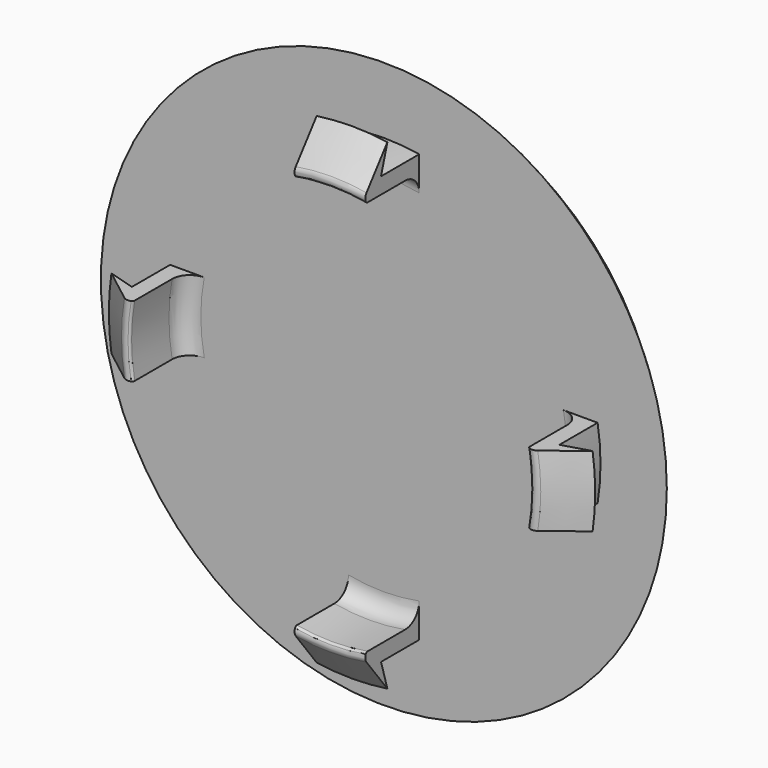
from build123d import *

# Parameters (mm, degrees)
F3_DEPTH      = 32.001
F3_DEPTH_BACK = 32.001
F5_DEPTH      = 32.001
F5_DEPTH_BACK = 32.001


# Not quite as in the source:
# - a feature names something its author has since deleted; it is built from what else it names


with BuildPart() as f1:
    # F0 (on Top) → F1 (revolve)
    with BuildSketch(Plane.XY):
        with BuildLine():
            Line((29, 3), (0, 3))
            Line((0, 3), (0, 0))
            Line((0, 0), (20.7, 0))
            ThreePointArc((20.7, 0), (22.1142135624, -0.5857864376), (22.7, -2))
            Line((22.7, -2), (22.7, -7.2844397868))
            ThreePointArc((22.7, -7.2844397868), (22.7497180358, -7.4498451628), (22.8823929227, -7.5604263361))
            ThreePointArc((22.8823929227, -7.5604263361), (23.3097624273, -7.6192211516), (23.7078530386, -7.45301228))
            Line((23.7078530386, -7.45301228), (27.5, -4.5))
            Line((27.5, -4.5), (24.5, -5.4))
            Line((24.5, -5.4), (24.5, -3))
            Line((24.5, -3), (24.5, 0))
            Line((24.5, 0), (32, 0))
            Line((32, 0), (29, 3))
        make_face()
    revolve(axis=Axis((0, -3.2623065636, 0), (0, -1, 0)))

    # F2 (on Top) → F3 (cut, two sides)
    with BuildSketch(Plane.XY) as f3_sk:
        with BuildLine():
            Line((-4, 0), (-18, 0))
            ThreePointArc((-18, 0), (-20.8284271247, -1.1715728753), (-22, -4))
            Line((-22, -4), (-22, -24.4516061772))
            Line((-22, -24.4516061772), (-4, -24.4516061772))
            Line((-4, -24.4516061772), (-4, 0))
        make_face()
        with BuildLine():
            Line((18, 0), (4, 0))
            Line((4, 0), (4, -24.4516061772))
            Line((4, -24.4516061772), (22, -24.4516061772))
            Line((22, -24.4516061772), (22, -4))
            ThreePointArc((22, -4), (20.8284271247, -1.1715728753), (18, 0))
        make_face()
    extrude(amount=-F3_DEPTH, mode=Mode.SUBTRACT)
    extrude(f3_sk.sketch, amount=F3_DEPTH_BACK, mode=Mode.SUBTRACT)

    # F4 (on Right) → F5 (cut, two sides)
    with BuildSketch(Plane.YZ) as f5_sk:
        with BuildLine():
            Line((-9.7492614017, 4), (0, 4))
            Line((0, 4), (0, 18))
            ThreePointArc((0, 18), (-1.1715728753, 20.8284271247), (-4, 22))
            Line((-4, 22), (-9.7492614017, 22))
            Line((-9.7492614017, 22), (-9.7492614017, 4))
        make_face()
        with BuildLine():
            Line((0, -18), (0, -4))
            Line((0, -4), (-9.764377423, -4))
            Line((-9.764377423, -4), (-9.764377423, -22))
            Line((-9.764377423, -22), (-4, -22))
            ThreePointArc((-4, -22), (-1.1715728753, -20.8284271247), (0, -18))
        make_face()
    extrude(amount=-F5_DEPTH, mode=Mode.SUBTRACT)
    extrude(f5_sk.sketch, amount=F5_DEPTH_BACK, mode=Mode.SUBTRACT)


solid = f1.part
